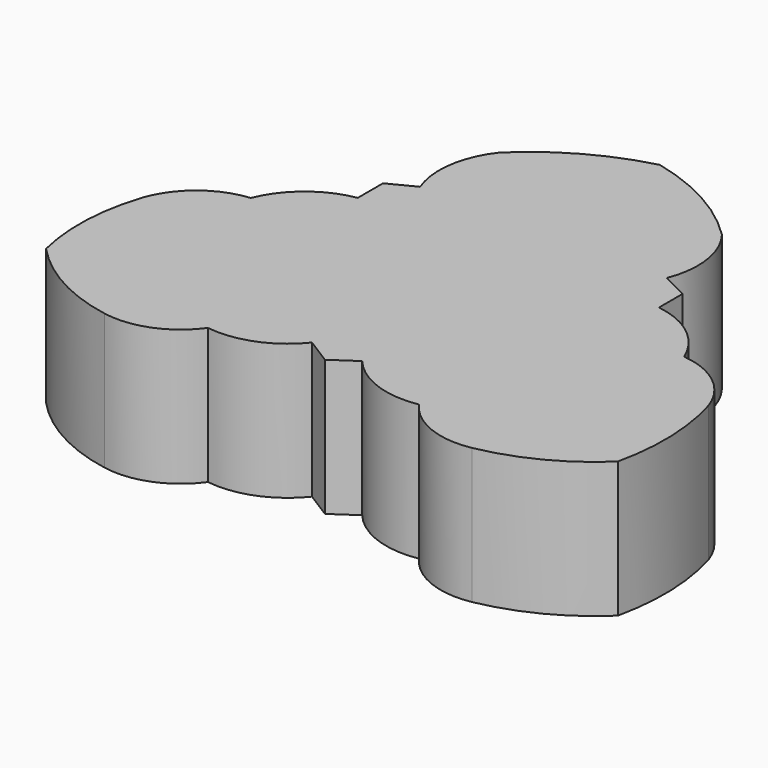
from build123d import *

# Parameters (mm, degrees)
F1_DEPTH = 11.1125


# Not quite as in the source:
# - a length typed as a fraction of an inch, garbled in the dataset ("3 / 203.2 mm" for 3/8 in), is restored


with BuildPart() as f1:
    # F0 (on Top) → F1 (new body)
    with BuildSketch(Plane.XY):
        with BuildLine():
            ThreePointArc((-0.1411418198, 20.1985444874), (-5.0054503986, 18.2564119782), (-9.2097157612, 15.1327075437))
            ThreePointArc((-9.2097157612, 15.1327075437), (-10.6205392688, 11.8246856933), (-10.2093555033, 8.2519613206))
            Line((-10.2093555033, 8.2519613206), (-12.369341217, 7.1464567445))
            Line((-12.369341217, 7.1464567445), (-12.369341217, 4.6386048198))
            Line((-12.369341217, 4.6386048198), (-12.369341217, 4.5682978211))
            ThreePointArc((-12.369341217, 4.5682978211), (-15.5930977879, 3.1185654947), (-17.7027139134, 0.2823972963))
            ThreePointArc((-17.7027139134, 0.2823972963), (-21.0452825194, -1.0603738309), (-23.1384971151, -3.9919692741))
            ThreePointArc((-23.1384971151, -3.9919692741), (-23.9954710425, -8.6613028545), (-23.5336683691, -13.3861117065))
            ThreePointArc((-23.5336683691, -13.3861117065), (-19.6562098094, -16.4130421994), (-15.0192606046, -18.054899429))
            ThreePointArc((-15.0192606046, -18.054899429), (-11.4338171794, -17.7079201351), (-8.5996589687, -15.484556372))
            ThreePointArc((-8.5996589687, -15.484556372), (-5.0294162563, -15.0523544446), (-2.1409380715, -12.9098966718))
            Line((-2.1409380715, -12.9098966718), (0, -14.2561570176))
            Line((0, -14.2561570176), (1.9696742658, -12.9098966718))
            ThreePointArc((1.9696742658, -12.9098966718), (4.9392756736, -15.0084468105), (8.560301624, -15.3410370587))
            ThreePointArc((8.560301624, -15.3410370587), (11.3944598347, -17.5644008218), (14.9799032599, -17.9113801157))
            ThreePointArc((14.9799032599, -17.9113801157), (19.5156578324, -16.3470620723), (23.423301056, -13.563092798))
            ThreePointArc((23.423301056, -13.563092798), (23.8861103651, -8.6849198531), (23.0991397704, -3.8484499608))
            ThreePointArc((23.0991397704, -3.8484499608), (21.0059251747, -0.9168545176), (17.6633565687, 0.4259166096))
            ThreePointArc((17.6633565687, 0.4259166096), (15.4847616458, 3.3168082822), (12.1560195839, 4.739132713))
            Line((12.1560195839, 4.739132713), (12.1560195839, 7.1464567445))
            Line((12.1560195839, 7.1464567445), (9.9960338703, 8.2519613206))
            ThreePointArc((9.9960338703, 8.2519613206), (10.4072176357, 11.8246856933), (8.9963941282, 15.1327075437))
            ThreePointArc((8.9963941282, 15.1327075437), (4.7823081966, 18.3053860292), (-0.1411418198, 20.1985444874))
        make_face()
    extrude(amount=F1_DEPTH)


solid = f1.part
